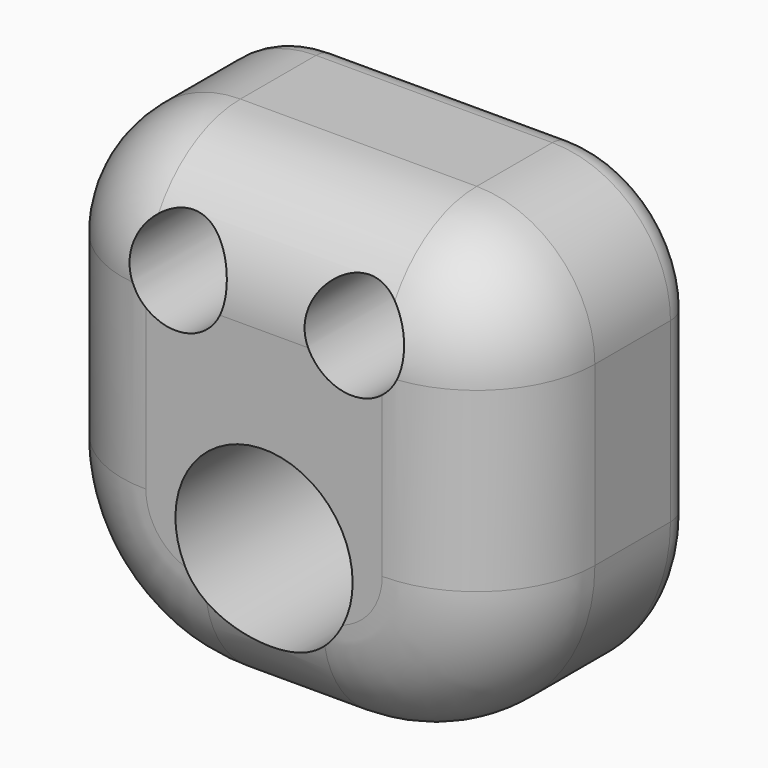
from build123d import *

# Parameters (mm, degrees)
F0_R         = 20.9202002185
F1_DEPTH     = 104.14
F2_T1_DEPTH  = 101.6
F2_T3_DEPTH  = 76.2
F2_T5_DEPTH  = 50.8
F2_T8_ANGLE  = 90
F2_T10_ANGLE = 90
F2_T12_ANGLE = 90
F2_T14_ANGLE = 90
F3_R         = 12.7
F4_R         = 38.1
F5_DEPTH     = 104.1410001


# Not quite as in the source:
# - a fillet or chamfer that OpenCascade refuses, or shapes differently, is made with other operations: its cross-section is extruded or revolved along the edge and cut away or added


with BuildPart() as f1:
    # F0 (on Front) → F1 (new body)
    with BuildSketch(Plane.XZ):
        with BuildLine():
            Line((0, 101.6), (-50.8, 101.6))
            ThreePointArc((-50.8, 101.6), (-86.7210244843, 86.7210244843), (-101.6, 50.8))
            Line((-101.6, 50.8), (-101.6, -25.4))
            ThreePointArc((-101.6, -25.4), (-79.2815367264, -79.2815367264), (-25.4, -101.6))
            Line((-25.4, -101.6), (0, -101.6))
            Line((0, -101.6), (0, 101.6))
        make_face()
        with Locations((-37.8764681518, 59.70396474)):
            Circle(F0_R, mode=Mode.SUBTRACT)
        with BuildLine():
            Line((50.8, 101.6), (0, 101.6))
            Line((0, 101.6), (0, -101.6))
            Line((0, -101.6), (25.4, -101.6))
            ThreePointArc((25.4, -101.6), (79.2815367264, -79.2815367264), (101.6, -25.4))
            Line((101.6, -25.4), (101.6, 50.8))
            ThreePointArc((101.6, 50.8), (86.7210244843, 86.7210244843), (50.8, 101.6))
        make_face()
        with Locations((37.8764681518, 59.70396474)):
            Circle(F0_R, mode=Mode.SUBTRACT)
    extrude(amount=F1_DEPTH)

    # F2: fillet of radius 50.8 on 1 edges, made by hand

    # F2_s2 → F2_t1 (cut)
    with BuildSketch(Plane.YZ.offset(-50.8)):
        with BuildLine():
            ThreePointArc((-53.34, 101.6), (-89.2610244843, 86.7210244843), (-104.14, 50.8))
            Line((-104.14, 50.8), (-104.14, 101.6))
            Line((-104.14, 101.6), (-53.34, 101.6))
        make_face()
    extrude(amount=F2_T1_DEPTH, mode=Mode.SUBTRACT)

    # F2_s4 → F2_t3 (cut)
    with BuildSketch(Plane.XY.offset(-25.4)):
        with BuildLine():
            ThreePointArc((-101.6, -53.34), (-86.7210244843, -89.2610244843), (-50.8, -104.14))
            Line((-50.8, -104.14), (-101.6, -104.14))
            Line((-101.6, -104.14), (-101.6, -53.34))
        make_face()
        with BuildLine():
            ThreePointArc((101.6, -53.34), (86.7210244843, -89.2610244843), (50.8, -104.14))
            Line((50.8, -104.14), (101.6, -104.14))
            Line((101.6, -104.14), (101.6, -53.34))
        make_face()
    extrude(amount=F2_T3_DEPTH, mode=Mode.SUBTRACT)

    # F2_s6 → F2_t5 (cut)
    with BuildSketch(Plane.YZ.offset(-25.4)):
        with BuildLine():
            ThreePointArc((-53.34, -101.6), (-89.2610244843, -86.7210244843), (-104.14, -50.8))
            Line((-104.14, -50.8), (-104.14, -101.6))
            Line((-104.14, -101.6), (-53.34, -101.6))
        make_face()
    extrude(amount=F2_T5_DEPTH, mode=Mode.SUBTRACT)

    # F2_s7 → F2_t8 (revolve, cut)
    with BuildSketch(Plane.YZ.offset(-50.8)):
        with BuildLine():
            ThreePointArc((-53.34, 101.6), (-89.2610244843, 86.7210244843), (-104.14, 50.8))
            Line((-104.14, 50.8), (-104.14, 101.6))
            Line((-104.14, 101.6), (-53.34, 101.6))
        make_face()
    revolve(axis=Axis((-50.8, -104.14, 50.8), (0, -1, 0)), revolution_arc=F2_T8_ANGLE, mode=Mode.SUBTRACT)

    # F2_s9 → F2_t10 (revolve, cut)
    with BuildSketch(Plane.XY.offset(-25.4)):
        with BuildLine():
            ThreePointArc((-101.6, -53.34), (-86.7210244843, -89.2610244843), (-50.8, -104.14))
            Line((-50.8, -104.14), (-101.6, -104.14))
            Line((-101.6, -104.14), (-101.6, -53.34))
        make_face()
    revolve(axis=Axis((-25.4, -104.14, -25.4), (0, -1, 0)), revolution_arc=F2_T10_ANGLE, mode=Mode.SUBTRACT)

    # F2_s11 → F2_t12 (revolve, cut)
    with BuildSketch(Plane.YZ.offset(25.4)):
        with BuildLine():
            ThreePointArc((-53.34, -101.6), (-89.2610244843, -86.7210244843), (-104.14, -50.8))
            Line((-104.14, -50.8), (-104.14, -101.6))
            Line((-104.14, -101.6), (-53.34, -101.6))
        make_face()
    revolve(axis=Axis((25.4, -104.14, -25.4), (0, -1, 0)), revolution_arc=F2_T12_ANGLE, mode=Mode.SUBTRACT)

    # F2_s13 → F2_t14 (revolve, cut)
    with BuildSketch(Plane.XY.offset(50.8)):
        with BuildLine():
            ThreePointArc((101.6, -53.34), (86.7210244843, -89.2610244843), (50.8, -104.14))
            Line((50.8, -104.14), (101.6, -104.14))
            Line((101.6, -104.14), (101.6, -53.34))
        make_face()
    revolve(axis=Axis((50.8, -104.14, 50.8), (0, -1, 0)), revolution_arc=F2_T14_ANGLE, mode=Mode.SUBTRACT)

    # F3
    f3_edges = [f1.edges().sort_by_distance(p)[0] for p in [
        (-86.721024, 0, 86.721024),
    ]]
    fillet(f3_edges, radius=F3_R)

    # F4 (on face) → F5 (cut, through all)
    with BuildSketch(Plane.XZ.offset(104.14)):
        with Locations((0, -31.9225803405)):
            Circle(F4_R)
    extrude(amount=-F5_DEPTH, mode=Mode.SUBTRACT)


solid = f1.part
